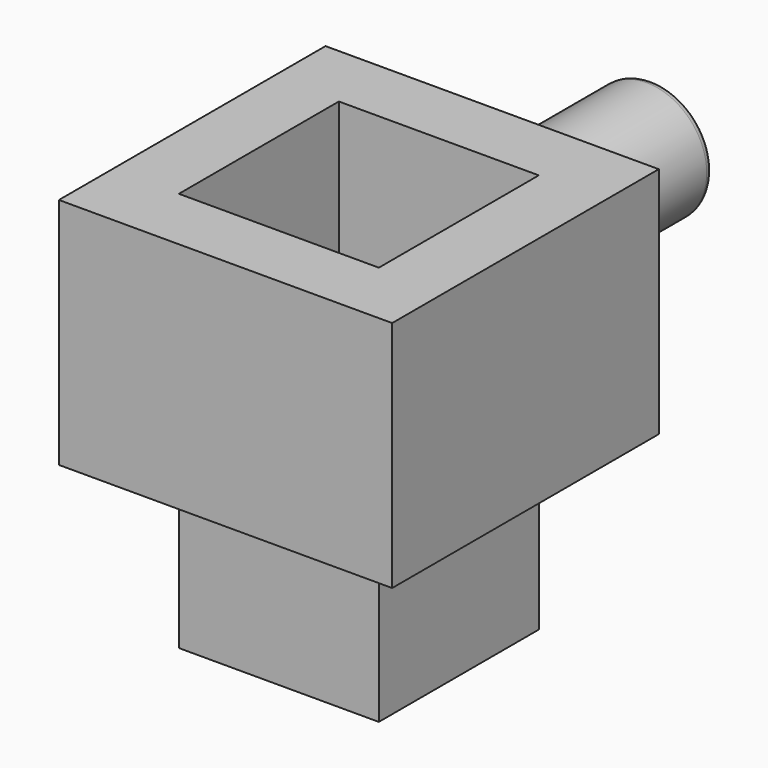
from build123d import *

# Parameters (mm, degrees)
F0_W     = 500
F0_H     = 500
F0_W_2   = 300
F0_H_2   = 300
F1_DEPTH = 350
F2_W     = 300
F2_H     = 300
F3_DEPTH = 250
F4_R     = 90
F4_R_2   = 75
F5_DEPTH = 300


# Not quite as in the source:
# - a fillet or chamfer that OpenCascade refuses, or shapes differently, is made with other operations: its cross-section is extruded or revolved along the edge and cut away or added


with BuildPart() as f1:
    # F0 (on Top) → F1 (new body)
    with BuildSketch(Plane.XY):
        with Locations((250, 250)):
            Rectangle(F0_W, F0_H)
        with Locations((250, 250)):
            Rectangle(F0_W_2, F0_H_2, mode=Mode.SUBTRACT)
    extrude(amount=F1_DEPTH)

    # F4 (on face) → F5 (join)
    with BuildSketch(Plane(origin=(0, 500, 0), x_dir=(-1, 0, 0), z_dir=(0, 1, 0))):
        with Locations((-250, 175)):
            Circle(F4_R)
        with Locations((-250, 175)):
            Circle(F4_R_2, mode=Mode.SUBTRACT)
    extrude(amount=F5_DEPTH)

    # F6: fillet of radius 10 on 3 edges, made by hand

    # F6_s1 → F6_t2 (revolve)
    with BuildSketch(Plane.XY.offset(175)):
        with BuildLine():
            add(Edge.make_bspline(
                [(150, 500), (160, 500), (160, 510)],
                knots=[0, 0, 0, 1, 1, 1], degree=2, weights=[1, 1, 1]))
            Line((160, 510), (160, 500))
            Line((160, 500), (150, 500))
        make_face()
    revolve(axis=Axis((250, 500, 175), (0, 1, 0)))

    # F6_s3 → F6_t4 (revolve, cut)
    with BuildSketch(Plane.XY.offset(175)):
        with BuildLine():
            add(Edge.make_bspline(
                [(160, 790), (160, 800), (170, 800)],
                knots=[0, 0, 0, 1, 1, 1], degree=2, weights=[1, 1, 1]))
            Line((170, 800), (160, 800))
            Line((160, 800), (160, 790))
        make_face()
    revolve(axis=Axis((250, 800, 175), (0, 1, 0)), mode=Mode.SUBTRACT)


with BuildPart() as f3:
    # F2 (on face) → F3 (new body)
    with BuildSketch(Plane(origin=(0, 0, 0), x_dir=(1, 0, 0), z_dir=(0, 0, -1))):
        with Locations((250, -250)):
            Rectangle(F2_W, F2_H)
    extrude(amount=F3_DEPTH)


solid = Compound([f1.part, f3.part])
